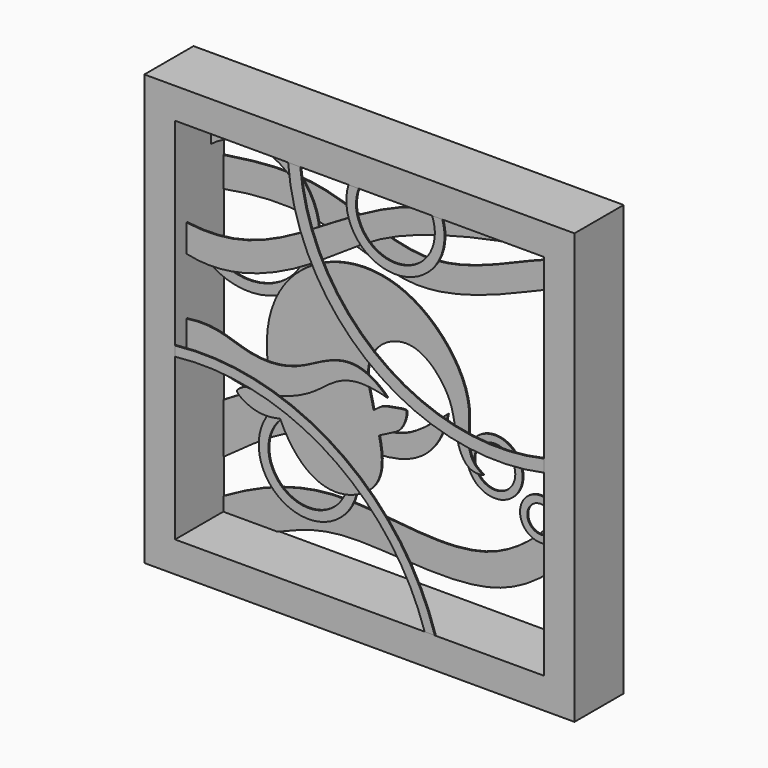
from build123d import *

# Parameters (mm, degrees)
F5_DEPTH  = 0.254
F6_W      = 88.9
F6_H      = 88.9
F6_W_2    = 76.2
F6_H_2    = 76.2
F7_DEPTH  = 12.7
F9_DEPTH  = 0.254
F8_R      = 5.7318385608
F8_R_2    = 4.2318385608
F8_R_3    = 4.2963833061
F8_R_4    = 2.7963833061
F8_R_5    = 10.2663851109
F8_R_6    = 8.2663851109
F11_DEPTH = 0.254
F13_DEPTH = 0.254
F15_DEPTH = 0.254


# Not quite as in the source:
# - a feature names something its author has since deleted; it is built from what else it names


with BuildPart() as f5:
    # F4 (on Front) → F5 (new body)
    with BuildSketch(Plane.XZ):
        with BuildLine():
            add(Edge.make_bspline(
                [(-38.1, 26.8125329167), (-32.3355323319, 27.6581205685), (-17.6620725027, 29.8550732727), (2.8911484909, 18.3366537215), (22.9848974303, 27.2909829997), (33.7973286493, 31.5962033457), (38.1, 31.9735445082)],
                knots=[0, 0, 0, 0, 0.2518954539, 0.5184541158, 0.7773202102, 1, 1, 1, 1], degree=3))
            Line((-38.1, 26.8125329167), (-38.1, 20.6539463252))
            add(Edge.make_bspline(
                [(-38.1, 20.6539463252), (-15.949960798, 24.7557926923), (-3.1076552532, 10.3004231639), (26.8026853229, 23.2868327058), (33.3267393056, 26.0228582677), (38.1, 27.3792054504)],
                knots=[0, 0, 0, 0, 0.421540471, 0.7603835902, 1, 1, 1, 1], degree=3))
            Line((38.1, 27.3792054504), (38.1, 31.9735445082))
        make_face()
    extrude(amount=F5_DEPTH)


with BuildPart() as f5b:
    # F4 (on Front) → F5, piece 2 (new body)
    with BuildSketch(Plane.XZ):
        with BuildLine():
            add(Edge.make_bspline(
                [(-38.1, -17.7561640739), (-33.6656508987, -14.8322757094), (-22.7778311537, -10.2528361771), (-2.8881114291, -13.9018176467), (2.204916316, -10.5626831297), (8.3523495123, -5.2179642953)],
                knots=[0, 0, 0, 0, 0.3374884851, 0.6843681215, 1, 1, 1, 1], degree=3))
            Line((-38.1, -17.7561640739), (-38.1, -28.1406063586))
            add(Edge.make_bspline(
                [(-38.1, -28.1406063586), (-32.8607403294, -24.5044174905), (-21.8896091488, -15.1759103778), (-1.227845599, -19.2927325329), (7.084956957, -12.1589361673), (8.3523495123, -5.2179642953)],
                knots=[0, 0, 0, 0, 0.3494949495, 0.6918172802, 1, 1, 1, 1], degree=3))
        make_face()
    extrude(amount=F5_DEPTH)


with BuildPart() as f5c:
    # F4 (on Front) → F5, piece 3 (new body)
    with BuildSketch(Plane.XZ):
        with BuildLine():
            Line((38.1, -17.1205457007), (38.1, -5.6588463485))
            add(Edge.make_bspline(
                [(-38.1, -35.2667570114), (-30.8100900765, -31.0820389991), (-14.7297369799, -24.3166769191), (19.0472567138, -34.1395350924), (33.6482086396, -14.5085496873), (38.1, -5.6588463485)],
                knots=[0, 0, 0, 0, 0.3106917137, 0.6579283948, 1, 1, 1, 1], degree=3))
            Line((-38.1, -35.2667570114), (-38.1, -38.1))
            Line((-38.1, -38.1), (-26.8868737349, -38.1))
            add(Edge.make_bspline(
                [(-26.8868737349, -38.1), (-22.9171591335, -36.4348137565), (-12.675325853, -32.0927122207), (20.0730540496, -38.8152516782), (33.3096922237, -23.9651451361), (38.1, -17.1205457007)],
                knots=[0, 0, 0, 0, 0.2642965298, 0.6486006357, 1, 1, 1, 1], degree=3))
        make_face()
    extrude(amount=F5_DEPTH)


with BuildPart() as f7:
    # F6 (on Front) → F7 (new body)
    with BuildSketch(Plane.XZ):
        Rectangle(F6_W, F6_H)
        Rectangle(F6_W_2, F6_H_2, mode=Mode.SUBTRACT)
    extrude(amount=F7_DEPTH)


with BuildPart() as f9:
    # F8 (on offset) → F9 (new body)
    with BuildSketch(Plane.XZ.offset(3.175)):
        with BuildLine():
            ThreePointArc((-38.1, 30.0955315868), (-17.7476064417, 20.3860998154), (-38.1, 10.676668044))
            Line((-38.1, 10.676668044), (-38.1, 8.0917770561))
            ThreePointArc((-38.1, 8.0917770561), (-15.6476064417, 20.3860998154), (-38.1, 32.6804225746))
            Line((-38.1, 32.6804225746), (-38.1, 30.0955315868))
        make_face()
    extrude(amount=F9_DEPTH)


with BuildPart() as f9b:
    # F8 (on offset) → F9, piece 2 (new body)
    with BuildSketch(Plane.XZ.offset(3.175)):
        with Locations((20.5689035356, -9.5632979646)):
            Circle(F8_R)
        with Locations((20.5689035356, -9.5632979646)):
            Circle(F8_R_2, mode=Mode.SUBTRACT)
    extrude(amount=F9_DEPTH)


with BuildPart() as f9c:
    # F8 (on offset) → F9, piece 3 (new body)
    with BuildSketch(Plane.XZ.offset(3.175)):
        with Locations((30.0695039332, -16.0241890699)):
            Circle(F8_R_3)
        with Locations((30.0695039332, -16.0241890699)):
            Circle(F8_R_4, mode=Mode.SUBTRACT)
    extrude(amount=F9_DEPTH)


with BuildPart() as f9d:
    # F8 (on offset) → F9, piece 4 (new body)
    with BuildSketch(Plane.XZ.offset(3.175)):
        with Locations((-17.9670006037, -21.3414989412)):
            Circle(F8_R_5)
        with Locations((-17.9670006037, -21.3414989412)):
            Circle(F8_R_6, mode=Mode.SUBTRACT)
    extrude(amount=F9_DEPTH)


with BuildPart() as f11:
    # F10 (on offset) → F11 (new body)
    with BuildSketch(Plane.XZ.offset(6.35)):
        with BuildLine():
            add(Edge.make_bspline(
                [(-6.4249184562, -22.1867698896), (-13.2500620283, -24.3848370363), (-18.3533044547, -19.5754182602), (-21.2606620079, -13.1306063645)],
                knots=[0, 0, 0, 0, 0.1494390843, 0.1494390843, 0.1494390843, 0.1494390843], degree=3))
            add(Edge.make_bspline(
                [(-6.4249184562, -22.1867698896), (0.3271782297, -19.6685342185), (0.3325228983, -14.6936954977), (-0.8361188761, -9.5263842392)],
                knots=[0, 0, 0, 0, 0.1658542317, 0.1658542317, 0.1658542317, 0.1658542317], degree=3))
            add(Edge.make_bspline(
                [(-0.8361188761, -9.5263842392), (-1.1549998819, -8.1164077627), (-1.5612901733, -6.6921007228), (-1.9417725248, -5.299461569)],
                knots=[0.1658542317, 0.1658542317, 0.1658542317, 0.1658542317, 0.2111099853, 0.2111099853, 0.2111099853, 0.2111099853], degree=3))
            add(Edge.make_bspline(
                [(-1.9417725248, -5.299461569), (-2.6000533519, -2.8900261501), (-4.6643068482, 5.3333283427), (5.7240046601, 11.9501215156), (13.4626363144, 3.4285478854), (14.7894718098, -1.4508946575), (16.2009540257, -10.7337011546), (20.7466702388, -9.7186805831)],
                knots=[0.2111099853, 0.2111099853, 0.2111099853, 0.2111099853, 0.2894079531, 0.4892832827, 0.6689639073, 0.8177799065, 1, 1, 1, 1], degree=3))
            add(Edge.make_bspline(
                [(-22.8413937426, -8.7478500813), (-23.5280594409, -6.2916352301), (-25.474620042, 6.0875369866), (-15.6571661637, 19.9634390542), (6.0761236204, 21.5467939449), (21.0755889091, 2.9836436132), (16.2009540257, -7.4482879276), (20.7466702388, -9.7186805831)],
                knots=[0.18194712, 0.18194712, 0.18194712, 0.18194712, 0.2351271942, 0.4436725558, 0.6389349958, 0.8438446644, 1, 1, 1, 1], degree=3))
            add(Edge.make_bspline(
                [(-21.2606620079, -13.1306063645), (-21.8931102289, -11.7286426421), (-22.4216471861, -10.2492906341), (-22.8413937426, -8.7478500813)],
                knots=[0.1494390843, 0.1494390843, 0.1494390843, 0.1494390843, 0.18194712, 0.18194712, 0.18194712, 0.18194712], degree=3))
        make_face()
        with BuildLine():
            add(Edge.make_bspline(
                [(-21.2606620079, -13.1306063645), (-23.9417216373, -13.766841494), (-27.0728004635, -13.4946693686), (-30.1745115386, -11.4744635518), (-30.1745115386, -10.9994667376)],
                knots=[0, 0, 0, 0, 0.5859832309, 1, 1, 1, 1], degree=3))
            add(Edge.make_bspline(
                [(-21.2606620079, -13.1306063645), (-21.8931102289, -11.7286426421), (-22.4216471861, -10.2492906341), (-22.8413937426, -8.7478500813)],
                knots=[0.1494390843, 0.1494390843, 0.1494390843, 0.1494390843, 0.18194712, 0.18194712, 0.18194712, 0.18194712], degree=3))
            add(Edge.make_bspline(
                [(-30.1745115386, -10.9994667376), (-30.2209632652, -10.4091996117), (-26.0324659486, -8.3973027584), (-25.0000113752, -8.9884115249), (-22.8413937426, -8.7478500813)],
                knots=[0, 0, 0, 0, 0.4946493079, 1, 1, 1, 1], degree=3))
        make_face()
        with BuildLine():
            add(Edge.make_bspline(
                [(-0.8361188761, -9.5263842392), (-1.1549998819, -8.1164077627), (-1.5612901733, -6.6921007228), (-1.9417725248, -5.299461569)],
                knots=[0.1658542317, 0.1658542317, 0.1658542317, 0.1658542317, 0.2111099853, 0.2111099853, 0.2111099853, 0.2111099853], degree=3))
            add(Edge.make_bspline(
                [(-0.8361188761, -9.5263842392), (1.7143883914, -8.0830363373), (3.9428798202, -7.7921529466), (5.0553672899, -3.841615334), (4.7971731499, -3.2698325001)],
                knots=[0, 0, 0, 0, 0.5571257635, 1, 1, 1, 1], degree=3))
            add(Edge.make_bspline(
                [(4.7971731499, -3.2698325001), (4.674169921, -2.9456391243), (0.9627219176, -3.816702895), (0, -3.6929372088), (-1.9417725248, -5.299461569)],
                knots=[0, 0, 0, 0, 0.4561308939, 1, 1, 1, 1], degree=3))
        make_face()
    extrude(amount=F11_DEPTH)


with BuildPart() as f13:
    # F12 (on offset) → F13 (new body)
    with BuildSketch(Plane.XZ.offset(9.525)):
        with BuildLine():
            Line((-38.1, 18.3793762699), (-38.1, 12.7131110057))
            add(Edge.make_bspline(
                [(-38.1, 12.7131110057), (-29.8648801095, 10.7582835795), (-12.8109966325, 17.4230931538), (2.0098964591, 30.4024004286), (25.9401214628, 36.1835043538), (31.1514478474, 36.851057469), (38.1, 36.4801175892)],
                knots=[0, 0, 0, 0, 0.2778110497, 0.5332891067, 0.7941499788, 1, 1, 1, 1], degree=3))
            Line((38.1, 36.4801175892), (38.1, 38.1))
            Line((38.1, 38.1), (15.5426803976, 38.1))
            add(Edge.make_bspline(
                [(-38.1, 18.3793762699), (-28.0447446464, 16.9817789183), (-12.4084848313, 24.4813999515), (4.2399876119, 36.3180371406), (15.5426803976, 38.1)],
                knots=[0, 0, 0, 0, 0.4776042611, 1, 1, 1, 1], degree=3))
        make_face()
    extrude(amount=F13_DEPTH)


with BuildPart() as f13b:
    # F12 (on offset) → F13, piece 2 (new body)
    with BuildSketch(Plane.XZ.offset(9.525)):
        with BuildLine():
            Line((-38.1, 0.8816549089), (-38.1, -5.7631321251))
            add(Edge.make_bspline(
                [(-38.1, -5.7631321251), (-33.37303248, -5.09123389), (-25.9376692324, -9.4116452168), (-10.0463203182, -4.6720105696), (-5.4601094794, 2.5368418346), (3.4122494981, 0)],
                knots=[0, 0, 0, 0, 0.316582736, 0.6491704703, 1, 1, 1, 1], degree=3))
            add(Edge.make_bspline(
                [(-38.1, 0.8816549089), (-32.2421744268, 1.8010044564), (-26.2678178426, -1.7193320409), (-13.6400698168, -1.7834828214), (-3.9446599055, 7.261102178), (3.4122494981, 0)],
                knots=[0, 0, 0, 0, 0.3194193715, 0.6204844796, 1, 1, 1, 1], degree=3))
        make_face()
    extrude(amount=F13_DEPTH)


with BuildPart() as f15:
    # F14 (on offset) → F15 (new body)
    with BuildSketch(Plane.XZ.offset(12.7)):
        with BuildLine():
            ThreePointArc((15.5667238507, -38.1), (-4.9006961689, -10.7770598292), (-38.1, -2.8231572042))
            Line((-38.1, -2.8231572042), (-38.1, -4.8361103178))
            ThreePointArc((-38.1, -4.8361103178), (-6.3494510194, -12.2203064086), (13.4713757063, -38.1))
            Line((13.4713757063, -38.1), (15.5667238507, -38.1))
        make_face()
    extrude(amount=-F15_DEPTH)


with BuildPart() as f15b:
    # F14 (on offset) → F15, piece 2 (new body)
    with BuildSketch(Plane.XZ.offset(12.7)):
        with BuildLine():
            Line((-12.2263851522, 38.1), (-14.7342916499, 38.1))
            ThreePointArc((-14.7342916499, 38.1), (2.7438206234, 6.4401517664), (38.1, -1.1605704824))
            Line((38.1, -1.1605704824), (38.1, 1.4023966748))
            ThreePointArc((38.1, 1.4023966748), (4.5334723431, 8.2270267426), (-12.2263851522, 38.1))
        make_face()
    extrude(amount=-F15_DEPTH)


with BuildPart() as f15c:
    # F14 (on offset) → F15, piece 3 (new body)
    with BuildSketch(Plane.XZ.offset(12.7)):
        with BuildLine():
            Line((-0.1382312425, 38.1), (-2.2558846455, 38.1))
            ThreePointArc((-2.2558846455, 38.1), (5.9318993208, 25.0796339249), (17.5889236284, 35.1137518883))
            ThreePointArc((17.5889236284, 35.1137518883), (17.4759520444, 36.6236866484), (17.1395528075, 38.1))
            Line((17.1395528075, 38.1), (15.0218994045, 38.1))
            ThreePointArc((15.0218994045, 38.1), (15.445912387, 36.6335540345), (15.5889236284, 35.1137518883))
            ThreePointArc((15.5889236284, 35.1137518883), (5.9220319347, 27.1096735822), (-0.1382312425, 38.1))
        make_face()
    extrude(amount=-F15_DEPTH)


solid = Compound([f5.part, f5b.part, f5c.part, f7.part, f9.part, f9b.part, f9c.part, f9d.part, f11.part, f13.part, f13b.part, f15.part, f15b.part, f15c.part])
